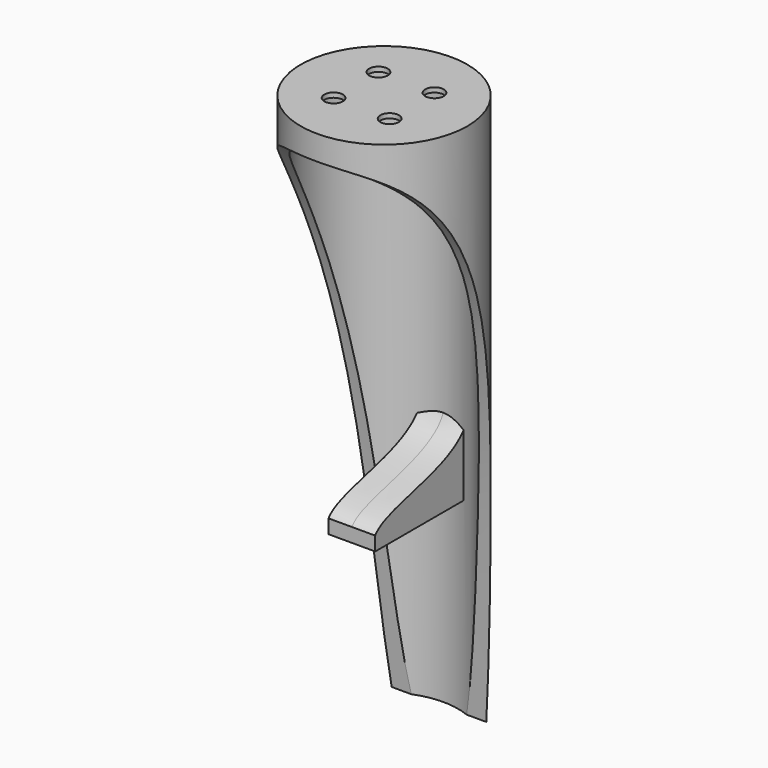
from build123d import *

# Parameters (mm, degrees)
F0_R      = 17.884061545
F1_DEPTH  = 1
F2_R      = 17.884061545
F2_R_2    = 15.884061545
F3_DEPTH  = 120
F5_DEPTH  = 100
F6_R      = 2
F7_DEPTH  = 121.0010007
F8_W      = 25
F8_H      = 3
F9_DEPTH  = 5
F10_R     = 1.6
F11_DEPTH = 2.5
F12_R     = 1
F13_DEPTH = 5


# Not quite as in the source:
# - a pattern or mirror of a feature is missing from the dataset's text; its kind, count and spacing are read off the source's solid
# - a feature names something its author has since deleted; it is built from what else it names


with BuildPart() as f1:
    # F0 (on Top) → F1 (new body)
    with BuildSketch(Plane.XY):
        Circle(F0_R)
    extrude(amount=F1_DEPTH)

    # F2 (on face) → F3 (join)
    with BuildSketch(Plane(origin=(0, 0, 0), x_dir=(1, 0, 0), z_dir=(0, 0, -1))):
        Circle(F2_R)
        Circle(F2_R_2, mode=Mode.SUBTRACT)
    extrude(amount=F3_DEPTH)

    # F4 (on Right) → F5 (cut, symmetric)
    with BuildSketch(Plane.YZ):
        with BuildLine():
            add(Edge.make_bspline(
                [(-23.545185104, -2.931100782), (-12.2797633222, -3.5261581086), (11.4767752963, -34.9586093489), (12.414609837, -94.1865478451), (15.1815395802, -125.3380775452)],
                knots=[0, 0, 0, 0, 0.3949910862, 1, 1, 1, 1], degree=3))
            Line((-23.545185104, -2.931100782), (-23.545185104, -130.5240243673))
            Line((-23.545185104, -130.5240243673), (15.1815395802, -125.3380775452))
        make_face()
    extrude(amount=F5_DEPTH, both=True, mode=Mode.SUBTRACT)

    # F6 (on face) → F7 (cut, through all)
    with BuildSketch(Plane.XY.offset(1)):
        with Locations((-6.0105, 6.0103152788)):
            Circle(F6_R)
        with Locations((6.0105, 6.0103152788)):
            Circle(F6_R)
        with Locations((6.0105, -6.0103152788)):
            Circle(F6_R)
        with Locations((-6.0105, -6.0103152788)):
            Circle(F6_R)
    extrude(amount=-F7_DEPTH, mode=Mode.SUBTRACT)

    # F8 (on Right) → F9 (join, symmetric)
    with BuildSketch(Plane.YZ):
        with BuildLine():
            Line((16.384061545, -77), (16.384061545, -63))
            add(Edge.make_bspline(
                [(16.384061545, -63), (16.384061545, -70), (-2.0563617415, -72.958536621), (-7.8631014511, -75.8217814094), (-8.615938455, -77)],
                knots=[0, 0, 0, 0, 0.622644618, 1, 1, 1, 1], degree=3))
            Line((-8.615938455, -77), (16.384061545, -77))
        make_face()
        with Locations((3.884061545, -78.5)):
            Rectangle(F8_W, F8_H)
    extrude(amount=F9_DEPTH, both=True)

    # F10 (on face) → F11 (join)
    with BuildSketch(Plane(origin=(0, 0, -80), x_dir=(1, 0, 0), z_dir=(0, 0, -1))):
        with Locations((0, -9.884061545)):
            Circle(F10_R)
    f11 = extrude(amount=F11_DEPTH)

    # F11_copies: F11 across plane
    add(f11.mirror(Plane(origin=(0, 3.634062, 0), x_dir=(0, 0, -1), z_dir=(0, -1, 0))))

    # F12 (on face) → F13 (cut)
    with BuildSketch(Plane(origin=(0, 0, -82.5), x_dir=(1, 0, 0), z_dir=(0, 0, -1))):
        with Locations((0, 2.615938455)):
            Circle(F12_R)
        with Locations((0, -9.884061545)):
            Circle(F12_R)
    extrude(amount=-F13_DEPTH, mode=Mode.SUBTRACT)


solid = f1.part
